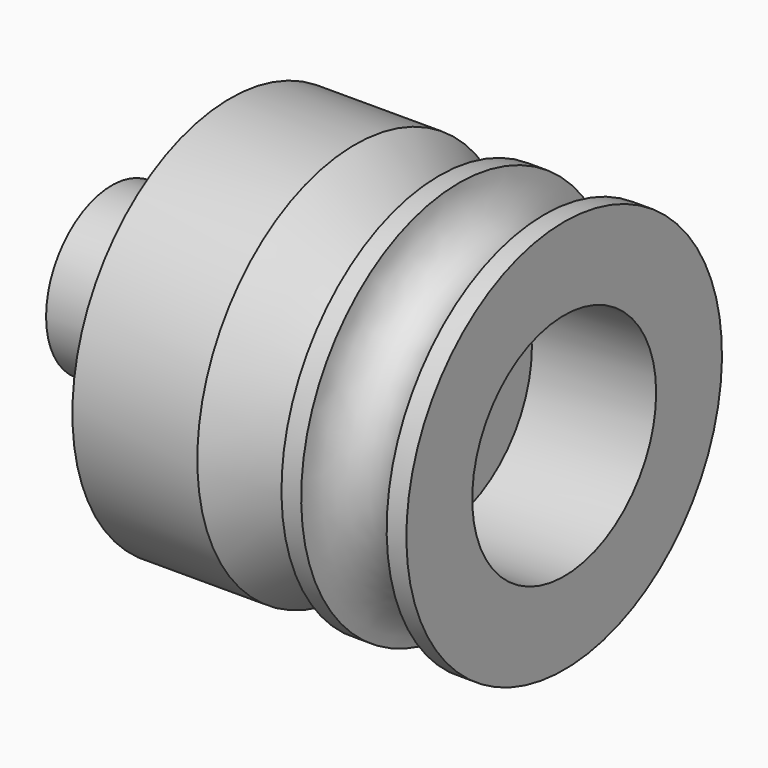
from build123d import *

# Parameters (mm, degrees)
F2_R      = 17.485
F3_DEPTH  = 18.9
F6_R      = 30
F4_R      = 18
F8_DEPTH  = 19
F9_R      = 12.5
F10_DEPTH = 18


with BuildPart() as f1:
    # F0 (on Front) → F1 (revolve)
    with BuildSketch(Plane.XZ):
        with BuildLine():
            Line((-12.1993720531, 30), (-12.1993720531, 0))
            Line((-12.1993720531, 0), (6.8006279469, 0))
            Line((6.8006279469, 0), (6.8006279469, 30))
            Line((6.8006279469, 30), (3.8006279469, 30))
            add(Edge.make_bspline(
                [(-9.1993720531, 30), (-9.1993720531, 23.015), (-2.6993720531, 23.015), (3.8006279469, 23.015), (3.8006279469, 30)],
                knots=[4.7123889804, 4.7123889804, 4.7123889804, 6.2831853072, 6.2831853072, 7.853981634, 7.853981634, 7.853981634], degree=2, weights=[1, 0.7071067812, 1, 0.7071067812, 1]))
            Line((-9.1993720531, 30), (-12.1993720531, 30))
        make_face()
    revolve(axis=Axis((-2.6993720531, 0, 0), (1, 0, 0)))

    # F2 (on face) → F3 (cut)
    with BuildSketch(Plane.YZ.offset(6.8006279469)):
        Circle(F2_R)
    extrude(amount=-F3_DEPTH, mode=Mode.SUBTRACT)

    # F6 (on offset) → F7 section 0
    with BuildSketch(Plane.YZ.offset(-25)):
        Circle(F6_R)
    # F4 (on face) → F7 section 1
    with BuildSketch(Plane(origin=(-12.1993720531, 0, 0), x_dir=(0, -1, 0), z_dir=(-1, 0, 0))):
        Circle(F4_R)
    loft()

    # F8 (add): a face of the model
    f8_faces = [f1.faces().sort_by_distance(p)[0] for p in [
        (-25, 0, 0),
    ]]
    extrude(f8_faces, amount=F8_DEPTH)

    # F9 (on face) → F10 (join)
    with BuildSketch(Plane(origin=(-44, 0, 0), x_dir=(0, -1, 0), z_dir=(-1, 0, 0))):
        Circle(F9_R)
    extrude(amount=F10_DEPTH)


solid = f1.part
